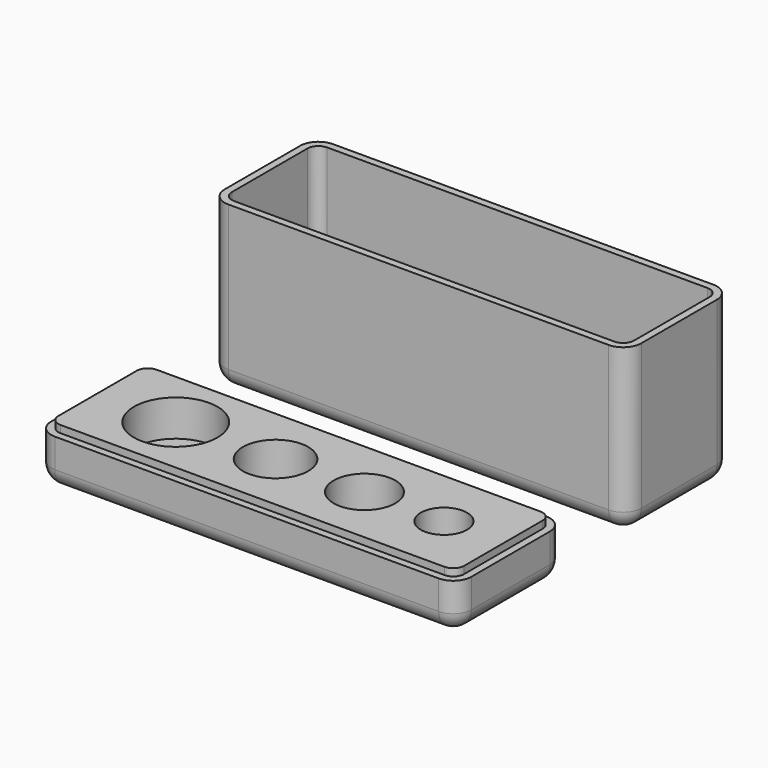
from build123d import *

# Parameters (mm, degrees)
F0_R          = 11.5
F1_DEPTH      = 5
F0_R_2        = 9
F0_R_3        = 8.5
F0_R_4        = 6.375
F0_W          = 115.75
F0_H          = 37
F0_W_2        = 111.75
F0_H_2        = 33
F2_DEPTH      = 13
F3_DEPTH      = 15
F4_W          = 110.75
F4_H          = 32
F5_DEPTH      = 2
F4_W_2        = 114.75
F4_H_2        = 36
F6_DEPTH      = 45
F7_R          = 5
F7_2_R        = 5
F8_R          = 3
F8_2_R        = 3
F10_T1_DEPTH  = 104.75
F10_S5_W      = 5
F10_S5_H      = 5
F10_T6_DEPTH  = 5
F10_S11_W     = 5
F10_S11_H     = 5
F10_T12_DEPTH = 5
F10_S17_W     = 5
F10_S17_H     = 5
F10_T18_DEPTH = 5
F10_S23_W     = 5
F10_S23_H     = 5
F10_T24_DEPTH = 5


# Not quite as in the source:
# - a fillet or chamfer that OpenCascade refuses, or shapes differently, is made with other operations: its cross-section is extruded or revolved along the edge and cut away or added


with BuildPart() as f1:
    # F0 (on Top) → F1 (new body)
    with BuildSketch(Plane.XY):
        with Locations((-34.375, 18.5)):
            Circle(F0_R)
    extrude(amount=F1_DEPTH)



with BuildPart() as f1b:
    # F0 (on Top) → F1, piece 2 (new body)
    with BuildSketch(Plane.XY):
        with Locations((-6.875, 18.5)):
            Circle(F0_R_2)
    extrude(amount=F1_DEPTH)


with BuildPart() as f1c:
    # F0 (on Top) → F1, piece 3 (new body)
    with BuildSketch(Plane.XY):
        with Locations((17.625, 18.5)):
            Circle(F0_R_3)
    extrude(amount=F1_DEPTH)


with BuildPart() as f1d:
    # F0 (on Top) → F1, piece 4 (new body)
    with BuildSketch(Plane.XY):
        with Locations((39.5, 18.5)):
            Circle(F0_R_4)
    extrude(amount=F1_DEPTH)


with BuildPart() as f2:
    # F0 (on Top) → F2 (new body)
    with BuildSketch(Plane.XY):
        with Locations((0, 18.5)):
            Rectangle(F0_W, F0_H)
        with Locations((0, 18.5)):
            Rectangle(F0_W_2, F0_H_2, mode=Mode.SUBTRACT)
    extrude(amount=F2_DEPTH)


with BuildPart() as f1_1:
    add(f1.part)

    add(f1b.part)  # F3 merges F1b

    add(f1c.part)  # F3 merges F1c

    add(f1d.part)  # F3 merges F1d

    add(f2.part)  # F3 merges F2
    # F0 (on Top) → F3 (join)
    with BuildSketch(Plane.XY):
        with Locations((0, 18.5)):
            Rectangle(F0_W_2, F0_H_2)
        with Locations((-34.375, 18.5)):
            Circle(F0_R, mode=Mode.SUBTRACT)
        with Locations((-6.875, 18.5)):
            Circle(F0_R_2, mode=Mode.SUBTRACT)
        with Locations((17.625, 18.5)):
            Circle(F0_R_3, mode=Mode.SUBTRACT)
        with Locations((39.5, 18.5)):
            Circle(F0_R_4, mode=Mode.SUBTRACT)
    extrude(amount=F3_DEPTH)

    # F7
    f7_edges = [f1_1.edges().sort_by_distance(p)[0] for p in [
        (-57.875, 37, 6.5),
        (-57.875, 0, 6.5),
        (57.875, 0, 6.5),
        (57.875, 37, 6.5),
        (0, 37, 0),
        (57.875, 18.5, 0),
        (0, 0, 0),
        (-57.875, 18.5, 0),
    ]]
    fillet(f7_edges, radius=F7_R)

    # F8
    f8_edges = [f1_1.edges().sort_by_distance(p)[0] for p in [
        (55.875, 35, 14),
        (55.875, 2, 14),
        (-55.875, 35, 14),
        (-55.875, 2, 14),
    ]]
    fillet(f8_edges, radius=F8_R)


with BuildPart() as f5:
    # F4 (on Top) → F5 (new body)
    with BuildSketch(Plane.XY):
        with Locations((-0.5, -22.2580123227)):
            Rectangle(F4_W, F4_H)
    extrude(amount=F5_DEPTH)

    # F4 (on Top) → F6 (join)
    with BuildSketch(Plane.XY):
        with Locations((-0.5, -22.2580123227)):
            Rectangle(F4_W_2, F4_H_2)
        with Locations((-0.5, -22.2580123227)):
            Rectangle(F4_W, F4_H, mode=Mode.SUBTRACT)
    extrude(amount=F6_DEPTH)

    # F7#2
    f7_2_edges = [f5.edges().sort_by_distance(p)[0] for p in [
        (56.875, -4.258012, 22.5),
        (56.875, -40.258012, 22.5),
        (-57.875, -4.258012, 22.5),
        (-57.875, -40.258012, 22.5),
        (-57.875, -22.258012, 0),
        (56.875, -22.258012, 0),
    ]]
    fillet(f7_2_edges, radius=F7_2_R)

    # F8#2
    f8_2_edges = [f5.edges().sort_by_distance(p)[0] for p in [
        (-55.875, -38.258012, 23.5),
        (-55.875, -6.258012, 23.5),
        (54.875, -38.258012, 23.5),
        (54.875, -6.258012, 23.5),
        (-0.5, -6.258012, 2),
        (-0.5, -38.258012, 2),
        (-55.875, -22.258012, 2),
        (54.875, -22.258012, 2),
    ]]
    fillet(f8_2_edges, radius=F8_2_R)


with BuildPart() as f5_1:
    # F9: moved
    add(f5.part.moved(Location((0, 100, 0))))

    # F10: fillet of radius 5 on 2 edges, made by hand

    # F10_s2 → F10_t1 (cut)
    with BuildSketch(Plane.YZ.offset(-52.875)):
        with BuildLine():
            ThreePointArc((95.7419876773, 5), (94.2775215832, 1.4644660941), (90.7419876773, 0))
            Line((90.7419876773, 0), (95.7419876773, 0))
            Line((95.7419876773, 0), (95.7419876773, 5))
        make_face()
        with BuildLine():
            ThreePointArc((59.7419876773, 5), (61.2064537714, 1.4644660941), (64.7419876773, 0))
            Line((64.7419876773, 0), (59.7419876773, 0))
            Line((59.7419876773, 0), (59.7419876773, 5))
        make_face()
    extrude(amount=F10_T1_DEPTH, mode=Mode.SUBTRACT)


with BuildPart() as f10_tool4:
    # F10_s5 → F10_t6 (new body)
    with BuildSketch(Plane.XZ.offset(-64.7419876773)):
        with Locations((-55.375, 2.5)):
            Rectangle(F10_S5_W, F10_S5_H)
    extrude(amount=F10_T6_DEPTH)

    # F10_s7 → F10_t8 (revolve, cut)
    with BuildSketch(Plane(origin=(-52.875, 64.7419876773, 5), x_dir=(0.7071067812, 0, 0.7071067812), z_dir=(0.7071067812, 0, -0.7071067812))):
        with BuildLine():
            ThreePointArc((0, -5), (5, 0), (0, 5))
            Line((0, 5), (0, -5))
        make_face()
    revolve(axis=Axis((-52.875, 64.7419876773, 5), (0, -1, 0)), mode=Mode.SUBTRACT)


with BuildPart() as f5_2:
    add(f5_1.part)

    # F10_t3: cut F10_tool4
    add(f10_tool4.part, mode=Mode.SUBTRACT)


with BuildPart() as f10_tool10:
    # F10_s11 → F10_t12 (new body)
    with BuildSketch(Plane.XZ.offset(-64.7419876773)):
        with Locations((54.375, 2.5)):
            Rectangle(F10_S11_W, F10_S11_H)
    extrude(amount=F10_T12_DEPTH)

    # F10_s13 → F10_t14 (revolve, cut)
    with BuildSketch(Plane(origin=(51.875, 64.7419876773, 5), x_dir=(-0.7071067812, 0, 0.7071067812), z_dir=(0.7071067812, 0, 0.7071067812))):
        with BuildLine():
            ThreePointArc((0, -5), (5, 0), (0, 5))
            Line((0, 5), (0, -5))
        make_face()
    revolve(axis=Axis((51.875, 64.7419876773, 5), (0, -1, 0)), mode=Mode.SUBTRACT)


with BuildPart() as f5_3:
    add(f5_2.part)

    # F10_t9: cut F10_tool10
    add(f10_tool10.part, mode=Mode.SUBTRACT)


with BuildPart() as f10_tool16:
    # F10_s17 → F10_t18 (new body)
    with BuildSketch(Plane.XZ.offset(-90.7419876773)):
        with Locations((54.375, 2.5)):
            Rectangle(F10_S17_W, F10_S17_H)
    extrude(amount=-F10_T18_DEPTH)

    # F10_s19 → F10_t20 (revolve, cut)
    with BuildSketch(Plane(origin=(51.875, 90.7419876773, 5), x_dir=(-0.7071067812, 0, 0.7071067812), z_dir=(-0.7071067812, 0, -0.7071067812))):
        with BuildLine():
            ThreePointArc((0, -5), (5, 0), (0, 5))
            Line((0, 5), (0, -5))
        make_face()
    revolve(axis=Axis((51.875, 90.7419876773, 5), (0, 1, 0)), mode=Mode.SUBTRACT)


with BuildPart() as f5_4:
    add(f5_3.part)

    # F10_t15: cut F10_tool16
    add(f10_tool16.part, mode=Mode.SUBTRACT)


with BuildPart() as f10_tool22:
    # F10_s23 → F10_t24 (new body)
    with BuildSketch(Plane.XZ.offset(-90.7419876773)):
        with Locations((-55.375, 2.5)):
            Rectangle(F10_S23_W, F10_S23_H)
    extrude(amount=-F10_T24_DEPTH)

    # F10_s25 → F10_t26 (revolve, cut)
    with BuildSketch(Plane(origin=(-52.875, 90.7419876773, 5), x_dir=(0.7071067812, 0, 0.7071067812), z_dir=(-0.7071067812, 0, 0.7071067812))):
        with BuildLine():
            ThreePointArc((0, -5), (5, 0), (0, 5))
            Line((0, 5), (0, -5))
        make_face()
    revolve(axis=Axis((-52.875, 90.7419876773, 5), (0, 1, 0)), mode=Mode.SUBTRACT)


with BuildPart() as f5_5:
    add(f5_4.part)

    # F10_t21: cut F10_tool22
    add(f10_tool22.part, mode=Mode.SUBTRACT)


solid = Compound([f1_1.part, f5_5.part])
